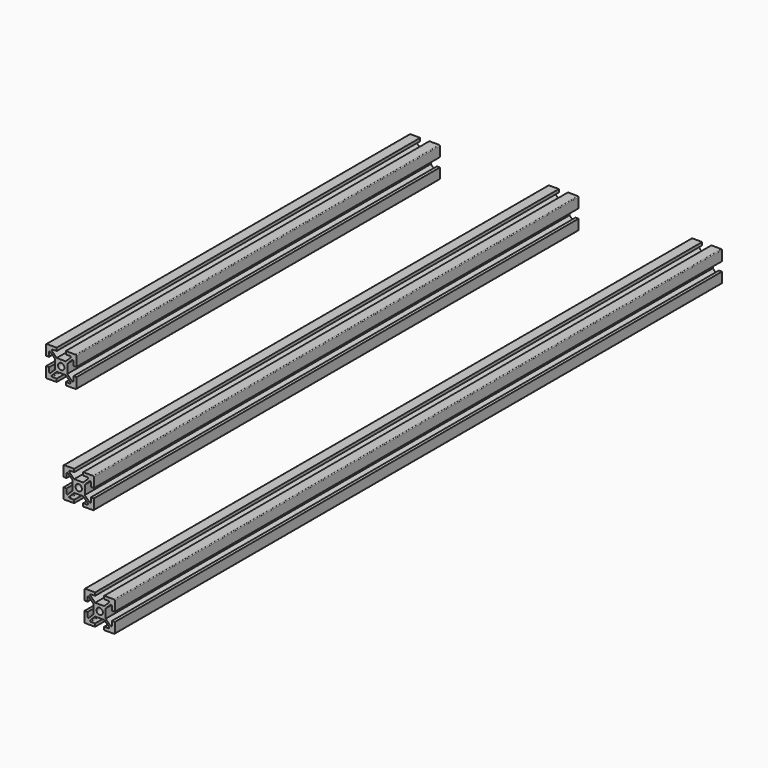
from build123d import *

# Parameters (mm, degrees)
F0_R     = 2.1
F1_DEPTH = 400
F2_DEPTH = 300
F3_DEPTH = 501


# Not quite as in the source:
# - ends of sketch curves that miss each other by under 0.0002 mm in the source are joined


with BuildPart() as f1:
    # F0 (on Front) → F1 (new body)
    with BuildSketch(Plane.XZ):
        with BuildLine():
            Line((-2.9999018588, 10), (-9.5002061197, 10))
            ThreePointArc((-9.5002061197, 10), (-9.8537595103, 9.8535533906), (-10.0002061197, 9.5))
            Line((-10.0002061197, 9.5), (-10.0000650851, 2.9996848913))
            Line((-10.0000650851, 2.9996848913), (-8.0000650797, 2.9997609984))
            Line((-8.0000650797, 2.9997609984), (-8.0001257238, 5.7948624374))
            ThreePointArc((-8.0001257238, 5.7948624374), (-7.6920243598, 6.2559885353), (-7.1480945067, 6.147803307))
            Line((-7.1480945067, 6.147803307), (-4.0000487303, 2.9998477851))
            Line((-4.0000487303, 2.9998477851), (-4.0000487303, -2.9998477851))
            Line((-4.0000487303, -2.9998477851), (-7.1480945067, -6.147803307))
            ThreePointArc((-7.1480945067, -6.147803307), (-7.6920243598, -6.2559885353), (-8.0001257238, -5.7948624374))
            Line((-8.0001257238, -5.7948624374), (-8.0000650797, -2.9997609984))
            Line((-8.0000650797, -2.9997609984), (-10.0000650851, -2.9996848913))
            Line((-10.0000650851, -2.9996848913), (-10.0002061194, -9.4999891517))
            ThreePointArc((-10.0002061194, -9.4999891517), (-9.8537595103, -9.8535533906), (-9.5002061197, -10))
            Line((-9.5002061197, -10), (-2.9999018588, -10))
            Line((-2.9999018588, -10), (-2.9999345728, -7.9999999934))
            Line((-2.9999345728, -7.9999999934), (-5.7950360114, -7.9999999934))
            ThreePointArc((-5.7950360114, -7.9999999934), (-6.2561554244, -7.6918886246), (-6.1479583947, -7.1479611189))
            Line((-6.1479583947, -7.1479611189), (-2.9999345717, -3.9999836431))
            Line((-2.9999345717, -3.9999836431), (2.9999345717, -3.9999836431))
            Line((2.9999345717, -3.9999836431), (6.1479583947, -7.1479611189))
            ThreePointArc((6.1479583947, -7.1479611189), (6.2561554244, -7.6918886246), (5.7950360114, -7.9999999934))
            Line((5.7950360114, -7.9999999934), (2.9999345728, -7.9999999934))
            Line((2.9999345728, -7.9999999934), (2.9999018588, -10))
            Line((2.9999018588, -10), (9.5002061197, -10))
            ThreePointArc((9.5002061197, -10), (9.8537595103, -9.8535533906), (10.0002061197, -9.5))
            Line((10.0002061197, -9.5), (10.0000650851, -2.9996848913))
            Line((10.0000650851, -2.9996848913), (8.0000650797, -2.9997609984))
            Line((8.0000650797, -2.9997609984), (8.0001257238, -5.7948624374))
            ThreePointArc((8.0001257238, -5.7948624374), (7.6920243598, -6.2559885353), (7.1480945067, -6.147803307))
            Line((7.1480945067, -6.147803307), (4.0000487303, -2.9998477851))
            Line((4.0000487303, -2.9998477851), (4.0000487303, 2.9998477851))
            Line((4.0000487303, 2.9998477851), (7.1480945067, 6.147803307))
            ThreePointArc((7.1480945067, 6.147803307), (7.6920243598, 6.2559885353), (8.0001257238, 5.7948624374))
            Line((8.0001257238, 5.7948624374), (8.0000650797, 2.9997609984))
            Line((8.0000650797, 2.9997609984), (10.0000650851, 2.9996848913))
            Line((10.0000650851, 2.9996848913), (10.0002061194, 9.4999891517))
            ThreePointArc((10.0002061194, 9.4999891517), (9.8537595103, 9.8535533906), (9.5002061197, 10))
            Line((9.5002061197, 10), (2.9999018588, 10))
            Line((2.9999018588, 10), (2.9999345728, 7.9999999934))
            Line((2.9999345728, 7.9999999934), (5.7950360114, 7.9999999934))
            ThreePointArc((5.7950360114, 7.9999999934), (6.2561554244, 7.6918886246), (6.1479583947, 7.1479611189))
            Line((6.1479583947, 7.1479611189), (2.9999345717, 3.9999836431))
            Line((2.9999345717, 3.9999836431), (-2.9999345717, 3.9999836431))
            Line((-2.9999345717, 3.9999836431), (-6.1479583947, 7.1479611189))
            ThreePointArc((-6.1479583947, 7.1479611189), (-6.2561554244, 7.6918886246), (-5.7950360114, 7.9999999934))
            Line((-5.7950360114, 7.9999999934), (-2.9999345728, 7.9999999934))
            Line((-2.9999345728, 7.9999999934), (-2.9999018588, 10))
        make_face()
        Circle(F0_R, mode=Mode.SUBTRACT)
    extrude(amount=F1_DEPTH)


with BuildPart() as f2:
    # F0 (on Front) → F2 (new body)
    with BuildSketch(Plane.XZ):
        with BuildLine():
            Line((-83.5317097726, 5.7948624374), (-83.5317704167, 2.9997609984))
            Line((-83.5317704167, 2.9997609984), (-81.5317704113, 2.9996848913))
            Line((-81.5317704113, 2.9996848913), (-81.531629377, 9.4999891517))
            ThreePointArc((-81.531629377, 9.4999891517), (-81.6780759861, 9.8535533906), (-82.0316293767, 10))
            Line((-82.0316293767, 10), (-88.5319336376, 10))
            Line((-88.5319336376, 10), (-88.5319009236, 7.9999999934))
            Line((-88.5319009236, 7.9999999934), (-85.736799485, 7.9999999934))
            ThreePointArc((-85.736799485, 7.9999999934), (-85.275680072, 7.6918886246), (-85.3838771017, 7.1479611189))
            Line((-85.3838771017, 7.1479611189), (-88.5319009247, 3.9999836431))
            Line((-88.5319009247, 3.9999836431), (-94.5317700681, 3.9999836431))
            Line((-94.5317700681, 3.9999836431), (-97.6797938911, 7.1479611189))
            ThreePointArc((-97.6797938911, 7.1479611189), (-97.7879909208, 7.6918886246), (-97.3268715078, 7.9999999934))
            Line((-97.3268715078, 7.9999999934), (-94.5317700692, 7.9999999934))
            Line((-94.5317700692, 7.9999999934), (-94.5317373552, 10))
            Line((-94.5317373552, 10), (-101.0320416161, 10))
            ThreePointArc((-101.0320416161, 10), (-101.3855950067, 9.8535533906), (-101.5320416161, 9.5))
            Line((-101.5320416161, 9.5), (-101.5319005815, 2.9996848913))
            Line((-101.5319005815, 2.9996848913), (-99.5319005761, 2.9997609984))
            Line((-99.5319005761, 2.9997609984), (-99.5319612202, 5.7948624374))
            ThreePointArc((-99.5319612202, 5.7948624374), (-99.2238598562, 6.2559885353), (-98.6799300032, 6.147803307))
            Line((-98.6799300032, 6.147803307), (-95.5318842267, 2.9998477851))
            Line((-95.5318842267, 2.9998477851), (-95.5318842267, -2.9998477851))
            Line((-95.5318842267, -2.9998477851), (-98.6799300032, -6.147803307))
            ThreePointArc((-98.6799300032, -6.147803307), (-99.2238598562, -6.2559885353), (-99.5319612202, -5.7948624374))
            Line((-99.5319612202, -5.7948624374), (-99.5319005761, -2.9997609984))
            Line((-99.5319005761, -2.9997609984), (-101.5319005815, -2.9996848913))
            Line((-101.5319005815, -2.9996848913), (-101.5320416159, -9.4999891517))
            ThreePointArc((-101.5320416159, -9.4999891517), (-101.3855950067, -9.8535533906), (-101.0320416161, -10))
            Line((-101.0320416161, -10), (-94.5317373552, -10))
            Line((-94.5317373552, -10), (-94.5317700692, -7.9999999934))
            Line((-94.5317700692, -7.9999999934), (-97.3268715078, -7.9999999934))
            ThreePointArc((-97.3268715078, -7.9999999934), (-97.7879909208, -7.6918886246), (-97.6797938911, -7.1479611189))
            Line((-97.6797938911, -7.1479611189), (-94.5317700681, -3.9999836431))
            Line((-94.5317700681, -3.9999836431), (-88.5319009247, -3.9999836431))
            Line((-88.5319009247, -3.9999836431), (-85.3838771017, -7.1479611189))
            ThreePointArc((-85.3838771017, -7.1479611189), (-85.275680072, -7.6918886246), (-85.736799485, -7.9999999934))
            Line((-85.736799485, -7.9999999934), (-88.5319009236, -7.9999999934))
            Line((-88.5319009236, -7.9999999934), (-88.5319336376, -10))
            Line((-88.5319336376, -10), (-82.0316293767, -10))
            ThreePointArc((-82.0316293767, -10), (-81.6780759861, -9.8535533906), (-81.5316293767, -9.5))
            Line((-81.5316293767, -9.5), (-81.5317704113, -2.9996848913))
            Line((-81.5317704113, -2.9996848913), (-83.5317704167, -2.9997609984))
            Line((-83.5317704167, -2.9997609984), (-83.5317097726, -5.7948624374))
            ThreePointArc((-83.5317097726, -5.7948624374), (-83.8398111366, -6.2559885353), (-84.3837409897, -6.147803307))
            Line((-84.3837409897, -6.147803307), (-87.5317867661, -2.9998477851))
            Line((-87.5317867661, -2.9998477851), (-87.5317867661, 2.9998477851))
            Line((-87.5317867661, 2.9998477851), (-84.3837409897, 6.147803307))
            ThreePointArc((-84.3837409897, 6.147803307), (-83.8398111366, 6.2559885353), (-83.5317097726, 5.7948624374))
        make_face()
        with Locations((-91.5318354964, 0)):
            Circle(F0_R, mode=Mode.SUBTRACT)
    extrude(amount=F2_DEPTH)


with BuildPart() as f3:
    # F0 (on Front) → F3 (new body)
    with BuildSketch(Plane.XZ):
        with BuildLine():
            Line((100.43342089, -7.9999999934), (97.6383194514, -7.9999999934))
            Line((97.6383194514, -7.9999999934), (97.6382867374, -10))
            Line((97.6382867374, -10), (104.1385909983, -10))
            ThreePointArc((104.1385909983, -10), (104.4921443889, -9.8535533906), (104.6385909983, -9.5))
            Line((104.6385909983, -9.5), (104.6384499637, -2.9996848913))
            Line((104.6384499637, -2.9996848913), (102.6384499583, -2.9997609984))
            Line((102.6384499583, -2.9997609984), (102.6385106025, -5.7948624374))
            ThreePointArc((102.6385106025, -5.7948624374), (102.3304092384, -6.2559885353), (101.7864793854, -6.147803307))
            Line((101.7864793854, -6.147803307), (98.638433609, -2.9998477851))
            Line((98.638433609, -2.9998477851), (98.638433609, 2.9998477851))
            Line((98.638433609, 2.9998477851), (101.7864793854, 6.147803307))
            ThreePointArc((101.7864793854, 6.147803307), (102.3304092384, 6.2559885353), (102.6385106025, 5.7948624374))
            Line((102.6385106025, 5.7948624374), (102.6384499583, 2.9997609984))
            Line((102.6384499583, 2.9997609984), (104.6384499637, 2.9996848913))
            Line((104.6384499637, 2.9996848913), (104.6385909981, 9.4999891517))
            ThreePointArc((104.6385909981, 9.4999891517), (104.4921443889, 9.8535533906), (104.1385909983, 10))
            Line((104.1385909983, 10), (97.6382867374, 10))
            Line((97.6382867374, 10), (97.6383194514, 7.9999999934))
            Line((97.6383194514, 7.9999999934), (100.43342089, 7.9999999934))
            ThreePointArc((100.43342089, 7.9999999934), (100.894540303, 7.6918886246), (100.7863432733, 7.1479611189))
            Line((100.7863432733, 7.1479611189), (97.6383194504, 3.9999836431))
            Line((97.6383194504, 3.9999836431), (91.6384503069, 3.9999836431))
            Line((91.6384503069, 3.9999836431), (88.4904264839, 7.1479611189))
            ThreePointArc((88.4904264839, 7.1479611189), (88.3822294542, 7.6918886246), (88.8433488673, 7.9999999934))
            Line((88.8433488673, 7.9999999934), (91.6384503058, 7.9999999934))
            Line((91.6384503058, 7.9999999934), (91.6384830198, 10))
            Line((91.6384830198, 10), (85.1381787589, 10))
            ThreePointArc((85.1381787589, 10), (84.7846253684, 9.8535533906), (84.6381787589, 9.5))
            Line((84.6381787589, 9.5), (84.6383197935, 2.9996848913))
            Line((84.6383197935, 2.9996848913), (86.6383197989, 2.9997609984))
            Line((86.6383197989, 2.9997609984), (86.6382591548, 5.7948624374))
            ThreePointArc((86.6382591548, 5.7948624374), (86.9463605188, 6.2559885353), (87.4902903719, 6.147803307))
            Line((87.4902903719, 6.147803307), (90.6383361483, 2.9998477851))
            Line((90.6383361483, 2.9998477851), (90.6383361483, -2.9998477851))
            Line((90.6383361483, -2.9998477851), (87.4902903719, -6.147803307))
            ThreePointArc((87.4902903719, -6.147803307), (86.9463605188, -6.2559885353), (86.6382591548, -5.7948624374))
            Line((86.6382591548, -5.7948624374), (86.6383197989, -2.9997609984))
            Line((86.6383197989, -2.9997609984), (84.6383197935, -2.9996848913))
            Line((84.6383197935, -2.9996848913), (84.6381787592, -9.4999891517))
            ThreePointArc((84.6381787592, -9.4999891517), (84.7846253684, -9.8535533906), (85.1381787589, -10))
            Line((85.1381787589, -10), (91.6384830198, -10))
            Line((91.6384830198, -10), (91.6384503058, -7.9999999934))
            Line((91.6384503058, -7.9999999934), (88.8433488673, -7.9999999934))
            ThreePointArc((88.8433488673, -7.9999999934), (88.3822294542, -7.6918886246), (88.4904264839, -7.1479611189))
            Line((88.4904264839, -7.1479611189), (91.6384503069, -3.9999836431))
            Line((91.6384503069, -3.9999836431), (97.6383194504, -3.9999836431))
            Line((97.6383194504, -3.9999836431), (100.7863432733, -7.1479611189))
            ThreePointArc((100.7863432733, -7.1479611189), (100.894540303, -7.6918886246), (100.43342089, -7.9999999934))
        make_face()
        with Locations((94.6383848786, 0)):
            Circle(F0_R, mode=Mode.SUBTRACT)
    extrude(amount=F3_DEPTH)


solid = Compound([f1.part, f2.part, f3.part])
